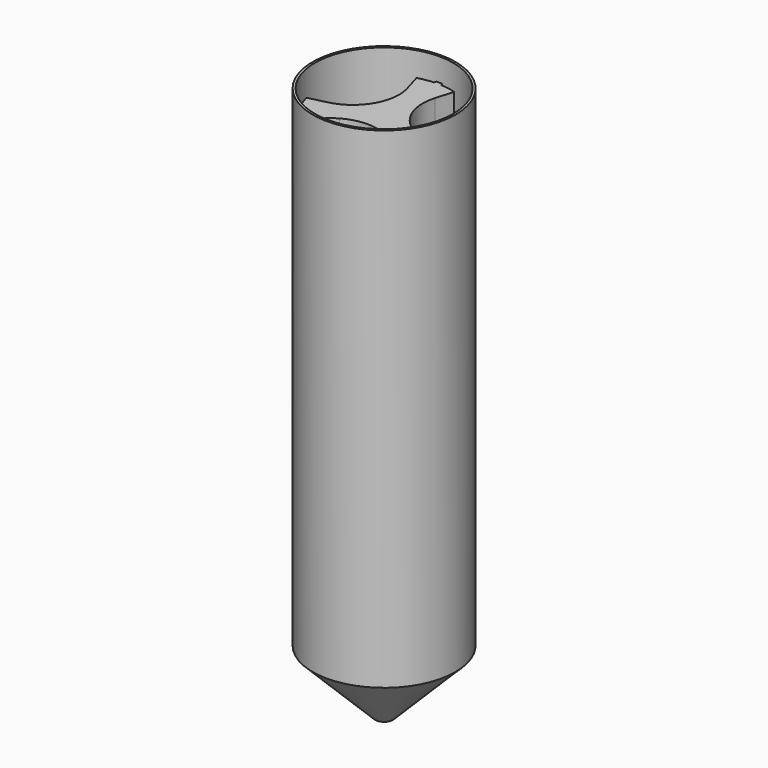
from build123d import *

# Parameters (mm, degrees)
F3_R            = 0.5
F4_DEPTH        = 25
F6_R            = 1.517812702
F7_DEPTH        = 25
F8_R            = 1.517812702
F9_DEPTH        = 25
F9_COPIES_COUNT = 3
F12_R           = 20.7909194511
F13_DEPTH       = 22


# Not quite as in the source:
# - a pattern or mirror of a feature is missing from the dataset's text; its kind, count and spacing are read off the source's solid


with BuildPart() as f1:
    # F0 (on Front) → F1 (revolve)
    with BuildSketch(Plane.XZ):
        Polygon((0, 0.5), (0, 0), (1.9198461069, 0), (15.5, 13.5801538931), (15.5, 120), (15, 120), (15, 13.5801538931), (1.9198461069, 0.5), align=None)
    revolve(axis=Axis((0, 0, 0.25), (0, 0, -1)))


with BuildPart() as f4:
    # F3 (on offset) → F4 (new body)
    with BuildSketch(Plane.XY.offset(50)):
        with BuildLine():
            ThreePointArc((12.9154450186, -6.5909999219), (14.0982969321, -3.38939871), (14.5, 0))
            ThreePointArc((14.5, 0), (10.5147839383, 9.9844538524), (0.7497491406, 14.4806034483))
            ThreePointArc((0.7497491406, 14.4806034483), (0, 13.75), (-0.7497491406, 14.4806034483))
            ThreePointArc((-0.7497491406, 14.4806034483), (-12.5573683549, 7.25), (-12.9154450186, -6.5909999219))
            ThreePointArc((-12.9154450186, -6.5909999219), (-12.1740000579, -6.6053848056), (-11.8073683549, -7.25))
            ThreePointArc((-11.8073683549, -7.25), (-11.9030540735, -7.6165689856), (-12.1656958781, -7.8896035263))
            ThreePointArc((-12.1656958781, -7.8896035263), (0, -14.5), (12.1656958781, -7.8896035263))
            ThreePointArc((12.1656958781, -7.8896035263), (11.907849302, -6.875), (12.9154450186, -6.5909999219))
        make_face()
        with Locations((-7.5, -7.5)):
            Circle(F3_R, mode=Mode.SUBTRACT)
        with Locations((7.5, -7.5)):
            Circle(F3_R, mode=Mode.SUBTRACT)
        with Locations((-7.5, 7.5)):
            Circle(F3_R, mode=Mode.SUBTRACT)
        with Locations((7.5, 7.5)):
            Circle(F3_R, mode=Mode.SUBTRACT)
        with BuildLine():
            ThreePointArc((-0.7497491406, 14.4806034483), (0, 13.75), (0.7497491406, 14.4806034483))
            ThreePointArc((0.7497491406, 14.4806034483), (0, 14.5), (-0.7497491406, 14.4806034483))
        make_face()
        with BuildLine():
            ThreePointArc((-0.7497491406, 14.4806034483), (0, 14.5), (0.7497491406, 14.4806034483))
            ThreePointArc((0.7497491406, 14.4806034483), (0.7499372825, 14.4903009131), (0.75, 14.5))
            ThreePointArc((0.75, 14.5), (-0.0096990869, 15.2499372825), (-0.7497491406, 14.4806034483))
        make_face()
        with BuildLine():
            ThreePointArc((13.3073683549, -7.25), (13.2019835493, -6.8666317031), (12.9154450186, -6.5909999219))
            ThreePointArc((12.9154450186, -6.5909999219), (12.5573683549, -7.25), (12.1656958781, -7.8896035263))
            ThreePointArc((12.1656958781, -7.8896035263), (12.9239373405, -7.9043142814), (13.3073683549, -7.25))
        make_face()
        with BuildLine():
            ThreePointArc((12.1656958781, -7.8896035263), (12.5573683549, -7.25), (12.9154450186, -6.5909999219))
            ThreePointArc((12.9154450186, -6.5909999219), (11.907849302, -6.875), (12.1656958781, -7.8896035263))
        make_face()
        with BuildLine():
            ThreePointArc((-11.8073683549, -7.25), (-12.1740000579, -6.6053848056), (-12.9154450186, -6.5909999219))
            ThreePointArc((-12.9154450186, -6.5909999219), (-12.5573683549, -7.25), (-12.1656958781, -7.8896035263))
            ThreePointArc((-12.1656958781, -7.8896035263), (-11.9030540735, -7.6165689856), (-11.8073683549, -7.25))
        make_face()
        with BuildLine():
            ThreePointArc((-12.1656958781, -7.8896035263), (-12.5573683549, -7.25), (-12.9154450186, -6.5909999219))
            ThreePointArc((-12.9154450186, -6.5909999219), (-13.2068874077, -7.625), (-12.1656958781, -7.8896035263))
        make_face()
    extrude(amount=F4_DEPTH)

    # F12 (on offset) → F13 (cut, through all)
    with BuildSketch(Plane.XY.offset(73.5)):
        Circle(F12_R)
        with BuildLine():
            ThreePointArc((12.1656958781, -7.8896035263), (0, -14.5), (-12.1656958781, -7.8896035263))
            ThreePointArc((-12.1656958781, -7.8896035263), (-4.1138430797, 13.9041826482), (14.5, 0))
            ThreePointArc((14.5, 0), (13.9041826482, -4.1138430797), (12.1656958781, -7.8896035263))
        make_face(mode=Mode.SUBTRACT)
    extrude(amount=-F13_DEPTH, mode=Mode.SUBTRACT)


with BuildPart() as f7:
    # F6 (on offset) → F7 (new body)
    with BuildSketch(Plane.XY.offset(90)):
        with BuildLine():
            ThreePointArc((12.9154450186, -6.5909999219), (12.5573683549, 7.25), (0.7497491406, 14.4806034483))
            ThreePointArc((0.7497491406, 14.4806034483), (0, 15.25), (-0.7497491406, 14.4806034483))
            ThreePointArc((-0.7497491406, 14.4806034483), (-12.5573683549, 7.25), (-12.9154450186, -6.5909999219))
            ThreePointArc((-12.9154450186, -6.5909999219), (-13.2068874077, -7.625), (-12.1656958781, -7.8896035263))
            ThreePointArc((-12.1656958781, -7.8896035263), (0, -14.5), (12.1656958781, -7.8896035263))
            ThreePointArc((12.1656958781, -7.8896035263), (13.2068874077, -7.625), (12.9154450186, -6.5909999219))
        make_face()
        with Locations((-7.5, 7.5)):
            Circle(F6_R, mode=Mode.SUBTRACT)
    extrude(amount=F7_DEPTH)

    # F8 (on face) → F9 (cut)
    with BuildSketch(Plane.XY.offset(115)):
        with BuildLine():
            ThreePointArc((-14.2644040621, -2.6032242994), (-12.5573683549, 7.25), (-4.877743656, 13.6549484373))
            ThreePointArc((-4.877743656, 13.6549484373), (-21.2176223927, 12.25), (-14.2644040621, -2.6032242994))
        make_face()
        with BuildLine():
            ThreePointArc((-10.2054687337, -2.4694942344), (-4.6986472053, 1.0661094856), (-2.5573683549, 7.25))
            ThreePointArc((-2.5573683549, 7.25), (-2.6595709496, 8.6760457652), (-2.9640896598, 10.072942415))
            ThreePointArc((-2.9640896598, 10.072942415), (-3.7371648595, 11.9621131459), (-4.877743656, 13.6549484373))
            ThreePointArc((-4.877743656, 13.6549484373), (-12.5573683549, 7.25), (-14.2644040621, -2.6032242994))
            ThreePointArc((-14.2644040621, -2.6032242994), (-12.2280762361, -2.7445768645), (-10.2054687337, -2.4694942344))
        make_face()
        with Locations((-7.5, 7.5)):
            Circle(F8_R, mode=Mode.SUBTRACT)
        with Locations((-7.5, 7.5)):
            Circle(F8_R)
        with BuildLine():
            ThreePointArc((-4.877743656, 13.6549484373), (-3.7371648595, 11.9621131459), (-2.9640896598, 10.072942415))
            Line((-2.9640896598, 10.072942415), (-4.0932667397, 13.9102540378))
            ThreePointArc((-4.0932667397, 13.9102540378), (-4.487321263, 13.7881814567), (-4.877743656, 13.6549484373))
        make_face()
        with BuildLine():
            Line((-14.0932667397, -3.4102540378), (-10.2054687337, -2.4694942344))
            ThreePointArc((-10.2054687337, -2.4694942344), (-12.2280762361, -2.7445768645), (-14.2644040621, -2.6032242994))
            ThreePointArc((-14.2644040621, -2.6032242994), (-14.184576045, -3.0079565196), (-14.0932667397, -3.4102540378))
        make_face()
    f9 = extrude(amount=-F9_DEPTH, mode=Mode.SUBTRACT)

    # F9_copies: F9 ×3 about axis
    f9_copies_axis = Axis((0, 0, 0), (0, 0, 1))
    for i in range(1, F9_COPIES_COUNT):
        add(f9.rotate(f9_copies_axis, i * 360 / F9_COPIES_COUNT), mode=Mode.SUBTRACT)


solid = Compound([f1.part, f4.part, f7.part])
